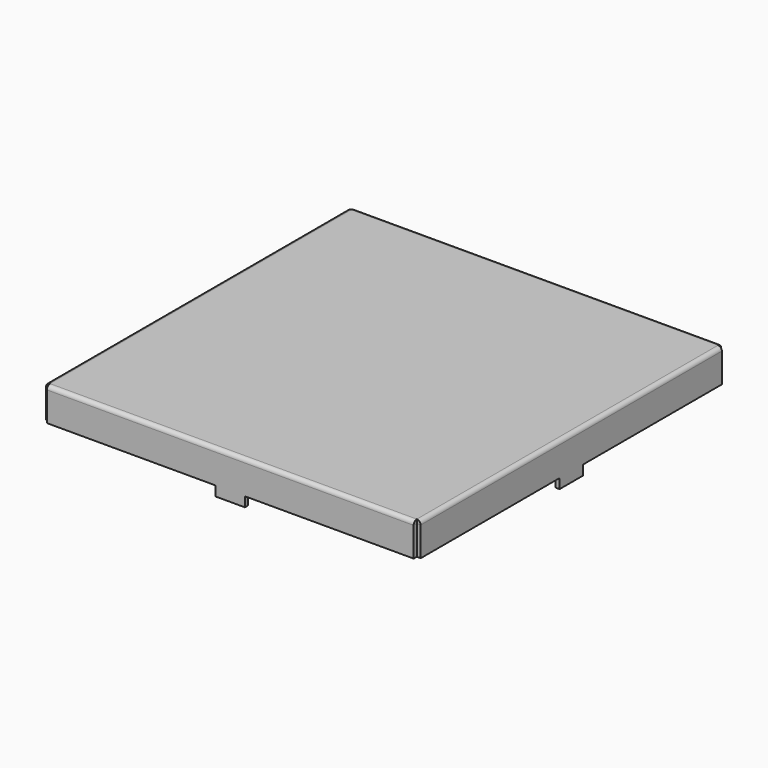
from build123d import *

# Parameters (mm, degrees)
F0_W     = 3.4
F0_H     = 0.2
F0_W_2   = 2
F0_W_3   = 0.85
F0_W_4   = 1.5
F0_W_5   = 11.05
F1_DEPTH = 1.5
F0_W_6   = 0.2
F0_H_2   = 8.9
F0_H_3   = 1.5
F2_DEPTH = 1.5
F3_DEPTH = 1.5
F0_W_7   = 8.65
F4_DEPTH = 1.5
F5_START = 1.5
F5_DEPTH = 0.2
F6_DEPTH = 0.7
F7_DEPTH = 0.5
F8_R     = 0.1999


# Not quite as in the source:
# - a fillet or chamfer is up to 0.001 mm smaller than in the source, because OpenCascade refuses the exact size


with BuildPart() as f1:
    # F0 (on Top) → F1 (new body)
    with BuildSketch(Plane.XY):
        with Locations((-7.7, 9.75)):
            Rectangle(F0_W, F0_H)
        with Locations((-5, 9.75)):
            Rectangle(F0_W_2, F0_H)
        with Locations((-3.575, 9.75)):
            Rectangle(F0_W_3, F0_H)
        with Locations((-2.4, 9.75)):
            Rectangle(F0_W_4, F0_H)
        with Locations((3.875, 9.75)):
            Rectangle(F0_W_5, F0_H)
    extrude(amount=F1_DEPTH)

    # F0 (on Top) → F6 (cut)
    with BuildSketch(Plane.XY):
        with Locations((-5, 9.75)):
            Rectangle(F0_W_2, F0_H)
    extrude(amount=F6_DEPTH, mode=Mode.SUBTRACT)

    # F0 (on Top) → F7 (join)
    with BuildSketch(Plane.XY):
        with Locations((-2.4, 9.75)):
            Rectangle(F0_W_4, F0_H)
    extrude(amount=-F7_DEPTH)


with BuildPart() as f2:
    # F0 (on Top) → F2 (new body)
    with BuildSketch(Plane.XY):
        with Locations((9.5, 5.2)):
            Rectangle(F0_W_6, F0_H_2)
        with Locations((9.5, 0)):
            Rectangle(F0_W_6, F0_H_3)
        with Locations((9.5, -5.2)):
            Rectangle(F0_W_6, F0_H_2)
    extrude(amount=F2_DEPTH)

    # F0 (on Top) → F7, piece 2 (join)
    with BuildSketch(Plane.XY):
        with Locations((9.5, 0)):
            Rectangle(F0_W_6, F0_H_3)
    extrude(amount=-F7_DEPTH)


with BuildPart() as f3:
    # F0 (on Top) → F3 (new body)
    with BuildSketch(Plane.XY):
        with Locations((-9.5, 5.2)):
            Rectangle(F0_W_6, F0_H_2)
        with Locations((-9.5, 0)):
            Rectangle(F0_W_6, F0_H_3)
        with Locations((-9.5, -5.2)):
            Rectangle(F0_W_6, F0_H_2)
    extrude(amount=F3_DEPTH)

    # F0 (on Top) → F7, piece 4 (join)
    with BuildSketch(Plane.XY):
        with Locations((-9.5, 0)):
            Rectangle(F0_W_6, F0_H_3)
    extrude(amount=-F7_DEPTH)


with BuildPart() as f4:
    # F0 (on Top) → F4 (new body)
    with BuildSketch(Plane.XY):
        with Locations((0, -9.75)):
            Rectangle(F0_W_4, F0_H)
        with Locations((5.075, -9.75)):
            Rectangle(F0_W_7, F0_H)
        with Locations((-5.075, -9.75)):
            Rectangle(F0_W_7, F0_H)
    extrude(amount=F4_DEPTH)

    # F0 (on Top) → F7, piece 3 (join)
    with BuildSketch(Plane.XY):
        with Locations((0, -9.75)):
            Rectangle(F0_W_4, F0_H)
    extrude(amount=-F7_DEPTH)


with BuildPart() as f5:
    # F0 (on Top) → F5 (new body)
    with BuildSketch(Plane.XY.offset(F5_START)):
        with Locations((-7.7, 9.75)):
            Rectangle(F0_W, F0_H)
        with Locations((-5, 9.75)):
            Rectangle(F0_W_2, F0_H)
        with Locations((-3.575, 9.75)):
            Rectangle(F0_W_3, F0_H)
        with Locations((-2.4, 9.75)):
            Rectangle(F0_W_4, F0_H)
        with Locations((3.875, 9.75)):
            Rectangle(F0_W_5, F0_H)
        with Locations((9.5, 5.2)):
            Rectangle(F0_W_6, F0_H_2)
        Polygon((9.4, 0.75), (9.4, 9.65), (-1.65, 9.65), (-3.15, 9.65), (-4, 9.65), (-6, 9.65), (-9.4, 9.65), (-9.4, 0.75), (-9.4, -0.75), (-9.4, -9.65), (-0.75, -9.65), (0.75, -9.65), (9.4, -9.65), (9.4, -0.75), align=None)
        with Locations((-9.5, 5.2)):
            Rectangle(F0_W_6, F0_H_2)
        with Locations((-9.5, 0)):
            Rectangle(F0_W_6, F0_H_3)
        with Locations((-9.5, -5.2)):
            Rectangle(F0_W_6, F0_H_2)
        with Locations((-5.075, -9.75)):
            Rectangle(F0_W_7, F0_H)
        with Locations((0, -9.75)):
            Rectangle(F0_W_4, F0_H)
        with Locations((5.075, -9.75)):
            Rectangle(F0_W_7, F0_H)
        with Locations((9.5, -5.2)):
            Rectangle(F0_W_6, F0_H_2)
        with Locations((9.5, 0)):
            Rectangle(F0_W_6, F0_H_3)
    extrude(amount=F5_DEPTH)

    # F8 (radius 0.2 in the source; OpenCascade refuses exactly that, so slightly less here)
    f8_edges = [f5.edges().sort_by_distance(p)[0] for p in [
        (-9.6, 0, 1.7),
        (0, 9.85, 1.7),
        (9.6, 0, 1.7),
        (0, -9.85, 1.7),
    ]]
    fillet(f8_edges, radius=F8_R)


solid = Compound([f1.part, f2.part, f3.part, f4.part, f5.part])
